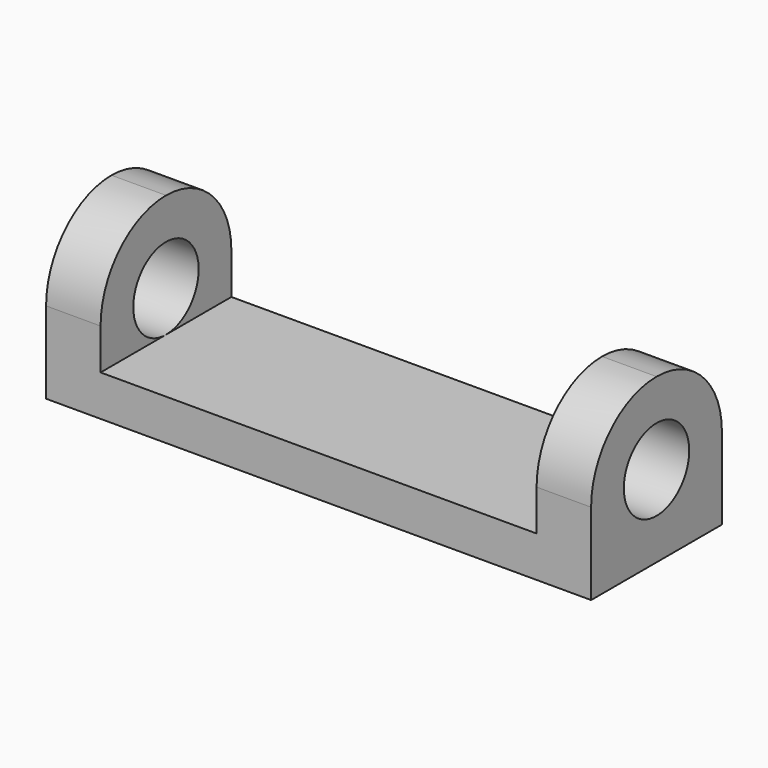
from build123d import *

# Parameters (mm, degrees)
F1_W     = 1
F1_H     = 3
F1_W_2   = 8
F2_DEPTH = 0.75
F3_DEPTH = 3
F4_R     = 0.75
F5_DEPTH = 10
F6_R     = 1.49999


# Not quite as in the source:
# - a fillet or chamfer is up to 0.001 mm smaller than in the source, because OpenCascade refuses the exact size


with BuildPart() as f2:
    # F1 (on Top) → F2 (new body)
    with BuildSketch(Plane.XY):
        with Locations((4.5, 0)):
            Rectangle(F1_W, F1_H)
        with Locations((-4.5, 0)):
            Rectangle(F1_W, F1_H)
        Rectangle(F1_W_2, F1_H)
    extrude(amount=F2_DEPTH)

    # F1 (on Top) → F3 (join)
    with BuildSketch(Plane.XY):
        with Locations((-4.5, 0)):
            Rectangle(F1_W, F1_H)
        with Locations((4.5, 0)):
            Rectangle(F1_W, F1_H)
    extrude(amount=F3_DEPTH)

    # F4 (on face) → F5 (cut, through all)
    with BuildSketch(Plane(origin=(-5, 0, 0), x_dir=(0, -1, 0), z_dir=(-1, 0, 0))):
        with Locations((0, 1.5)):
            Circle(F4_R)
    extrude(amount=-F5_DEPTH, mode=Mode.SUBTRACT)

    # F6 (radius 1.5 in the source; OpenCascade refuses exactly that, so slightly less here)
    f6_edges = [f2.edges().sort_by_distance(p)[0] for p in [
        (4.5, 1.5, 3),
        (4.5, -1.5, 3),
        (-4.5, -1.5, 3),
        (-4.5, 1.5, 3),
    ]]
    fillet(f6_edges, radius=F6_R)


solid = f2.part
